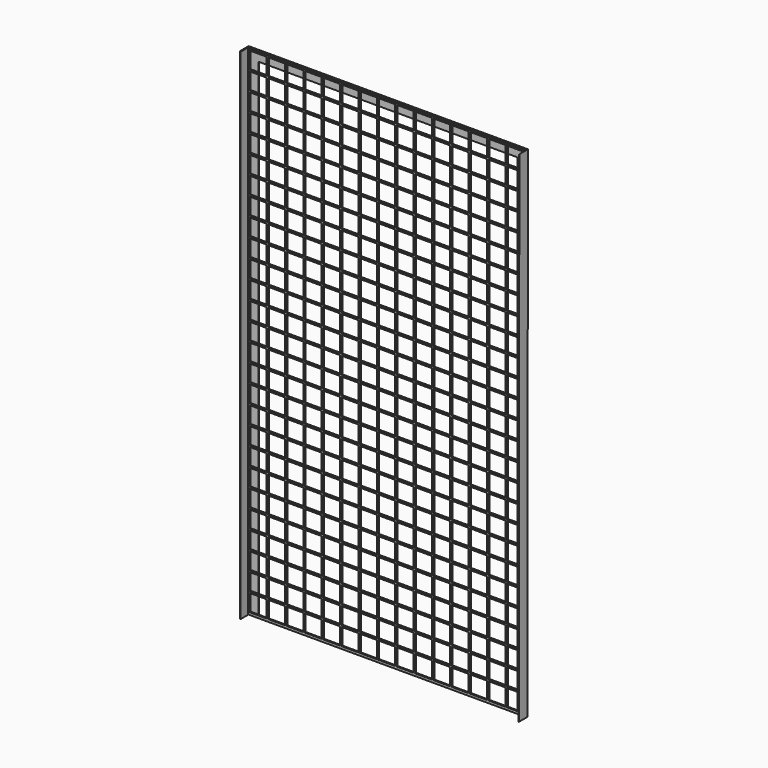
from build123d import *

# Parameters (mm, degrees)
F0_W     = 815
F0_H     = 1465
F0_W_2   = 50
F0_H_2   = 50
F1_DEPTH = 4
F3_DEPTH = 1.5
F4_DEPTH = 30


with BuildPart() as f1:
    # F0 (on Front) → F1 (new body)
    with BuildSketch(Plane.XZ):
        with Locations((407.5, -732.5)):
            Rectangle(F0_W, F0_H)
        with Locations((29, -1433)):
            Rectangle(F0_W_2, F0_H_2, mode=Mode.SUBTRACT)
        with Locations((29, -1379)):
            Rectangle(F0_W_2, F0_H_2, mode=Mode.SUBTRACT)
        with Locations((83, -1433)):
            Rectangle(F0_W_2, F0_H_2, mode=Mode.SUBTRACT)
        with Locations((83, -1379)):
            Rectangle(F0_W_2, F0_H_2, mode=Mode.SUBTRACT)
        with Locations((29, -1325)):
            Rectangle(F0_W_2, F0_H_2, mode=Mode.SUBTRACT)
        with Locations((83, -1325)):
            Rectangle(F0_W_2, F0_H_2, mode=Mode.SUBTRACT)
        with Locations((137, -1433)):
            Rectangle(F0_W_2, F0_H_2, mode=Mode.SUBTRACT)
        with Locations((137, -1379)):
            Rectangle(F0_W_2, F0_H_2, mode=Mode.SUBTRACT)
        with Locations((191, -1433)):
            Rectangle(F0_W_2, F0_H_2, mode=Mode.SUBTRACT)
        with Locations((191, -1379)):
            Rectangle(F0_W_2, F0_H_2, mode=Mode.SUBTRACT)
        with Locations((137, -1325)):
            Rectangle(F0_W_2, F0_H_2, mode=Mode.SUBTRACT)
        with Locations((191, -1325)):
            Rectangle(F0_W_2, F0_H_2, mode=Mode.SUBTRACT)
        with Locations((29, -1271)):
            Rectangle(F0_W_2, F0_H_2, mode=Mode.SUBTRACT)
        with Locations((29, -1217)):
            Rectangle(F0_W_2, F0_H_2, mode=Mode.SUBTRACT)
        with Locations((83, -1271)):
            Rectangle(F0_W_2, F0_H_2, mode=Mode.SUBTRACT)
        with Locations((83, -1217)):
            Rectangle(F0_W_2, F0_H_2, mode=Mode.SUBTRACT)
        with Locations((29, -1163)):
            Rectangle(F0_W_2, F0_H_2, mode=Mode.SUBTRACT)
        with Locations((29, -1109)):
            Rectangle(F0_W_2, F0_H_2, mode=Mode.SUBTRACT)
        with Locations((83, -1163)):
            Rectangle(F0_W_2, F0_H_2, mode=Mode.SUBTRACT)
        with Locations((83, -1109)):
            Rectangle(F0_W_2, F0_H_2, mode=Mode.SUBTRACT)
        with Locations((137, -1271)):
            Rectangle(F0_W_2, F0_H_2, mode=Mode.SUBTRACT)
        with Locations((137, -1217)):
            Rectangle(F0_W_2, F0_H_2, mode=Mode.SUBTRACT)
        with Locations((191, -1271)):
            Rectangle(F0_W_2, F0_H_2, mode=Mode.SUBTRACT)
        with Locations((191, -1217)):
            Rectangle(F0_W_2, F0_H_2, mode=Mode.SUBTRACT)
        with Locations((137, -1163)):
            Rectangle(F0_W_2, F0_H_2, mode=Mode.SUBTRACT)
        with Locations((137, -1109)):
            Rectangle(F0_W_2, F0_H_2, mode=Mode.SUBTRACT)
        with Locations((191, -1163)):
            Rectangle(F0_W_2, F0_H_2, mode=Mode.SUBTRACT)
        with Locations((191, -1109)):
            Rectangle(F0_W_2, F0_H_2, mode=Mode.SUBTRACT)
        with Locations((245, -1433)):
            Rectangle(F0_W_2, F0_H_2, mode=Mode.SUBTRACT)
        with Locations((245, -1379)):
            Rectangle(F0_W_2, F0_H_2, mode=Mode.SUBTRACT)
        with Locations((299, -1433)):
            Rectangle(F0_W_2, F0_H_2, mode=Mode.SUBTRACT)
        with Locations((299, -1379)):
            Rectangle(F0_W_2, F0_H_2, mode=Mode.SUBTRACT)
        with Locations((245, -1325)):
            Rectangle(F0_W_2, F0_H_2, mode=Mode.SUBTRACT)
        with Locations((299, -1325)):
            Rectangle(F0_W_2, F0_H_2, mode=Mode.SUBTRACT)
        with Locations((353, -1433)):
            Rectangle(F0_W_2, F0_H_2, mode=Mode.SUBTRACT)
        with Locations((353, -1379)):
            Rectangle(F0_W_2, F0_H_2, mode=Mode.SUBTRACT)
        with Locations((407, -1433)):
            Rectangle(F0_W_2, F0_H_2, mode=Mode.SUBTRACT)
        with Locations((407, -1379)):
            Rectangle(F0_W_2, F0_H_2, mode=Mode.SUBTRACT)
        with Locations((353, -1325)):
            Rectangle(F0_W_2, F0_H_2, mode=Mode.SUBTRACT)
        with Locations((407, -1325)):
            Rectangle(F0_W_2, F0_H_2, mode=Mode.SUBTRACT)
        with Locations((245, -1271)):
            Rectangle(F0_W_2, F0_H_2, mode=Mode.SUBTRACT)
        with Locations((245, -1217)):
            Rectangle(F0_W_2, F0_H_2, mode=Mode.SUBTRACT)
        with Locations((299, -1271)):
            Rectangle(F0_W_2, F0_H_2, mode=Mode.SUBTRACT)
        with Locations((299, -1217)):
            Rectangle(F0_W_2, F0_H_2, mode=Mode.SUBTRACT)
        with Locations((245, -1163)):
            Rectangle(F0_W_2, F0_H_2, mode=Mode.SUBTRACT)
        with Locations((245, -1109)):
            Rectangle(F0_W_2, F0_H_2, mode=Mode.SUBTRACT)
        with Locations((299, -1163)):
            Rectangle(F0_W_2, F0_H_2, mode=Mode.SUBTRACT)
        with Locations((299, -1109)):
            Rectangle(F0_W_2, F0_H_2, mode=Mode.SUBTRACT)
        with Locations((353, -1271)):
            Rectangle(F0_W_2, F0_H_2, mode=Mode.SUBTRACT)
        with Locations((353, -1217)):
            Rectangle(F0_W_2, F0_H_2, mode=Mode.SUBTRACT)
        with Locations((407, -1271)):
            Rectangle(F0_W_2, F0_H_2, mode=Mode.SUBTRACT)
        with Locations((407, -1217)):
            Rectangle(F0_W_2, F0_H_2, mode=Mode.SUBTRACT)
        with Locations((353, -1163)):
            Rectangle(F0_W_2, F0_H_2, mode=Mode.SUBTRACT)
        with Locations((353, -1109)):
            Rectangle(F0_W_2, F0_H_2, mode=Mode.SUBTRACT)
        with Locations((407, -1163)):
            Rectangle(F0_W_2, F0_H_2, mode=Mode.SUBTRACT)
        with Locations((407, -1109)):
            Rectangle(F0_W_2, F0_H_2, mode=Mode.SUBTRACT)
        with Locations((29, -1055)):
            Rectangle(F0_W_2, F0_H_2, mode=Mode.SUBTRACT)
        with Locations((83, -1055)):
            Rectangle(F0_W_2, F0_H_2, mode=Mode.SUBTRACT)
        with Locations((29, -1001)):
            Rectangle(F0_W_2, F0_H_2, mode=Mode.SUBTRACT)
        with Locations((29, -947)):
            Rectangle(F0_W_2, F0_H_2, mode=Mode.SUBTRACT)
        with Locations((83, -1001)):
            Rectangle(F0_W_2, F0_H_2, mode=Mode.SUBTRACT)
        with Locations((83, -947)):
            Rectangle(F0_W_2, F0_H_2, mode=Mode.SUBTRACT)
        with Locations((137, -1055)):
            Rectangle(F0_W_2, F0_H_2, mode=Mode.SUBTRACT)
        with Locations((191, -1055)):
            Rectangle(F0_W_2, F0_H_2, mode=Mode.SUBTRACT)
        with Locations((137, -1001)):
            Rectangle(F0_W_2, F0_H_2, mode=Mode.SUBTRACT)
        with Locations((137, -947)):
            Rectangle(F0_W_2, F0_H_2, mode=Mode.SUBTRACT)
        with Locations((191, -1001)):
            Rectangle(F0_W_2, F0_H_2, mode=Mode.SUBTRACT)
        with Locations((191, -947)):
            Rectangle(F0_W_2, F0_H_2, mode=Mode.SUBTRACT)
        with Locations((29, -893)):
            Rectangle(F0_W_2, F0_H_2, mode=Mode.SUBTRACT)
        with Locations((29, -839)):
            Rectangle(F0_W_2, F0_H_2, mode=Mode.SUBTRACT)
        with Locations((83, -893)):
            Rectangle(F0_W_2, F0_H_2, mode=Mode.SUBTRACT)
        with Locations((83, -839)):
            Rectangle(F0_W_2, F0_H_2, mode=Mode.SUBTRACT)
        with Locations((29, -785)):
            Rectangle(F0_W_2, F0_H_2, mode=Mode.SUBTRACT)
        with Locations((83, -785)):
            Rectangle(F0_W_2, F0_H_2, mode=Mode.SUBTRACT)
        with Locations((137, -893)):
            Rectangle(F0_W_2, F0_H_2, mode=Mode.SUBTRACT)
        with Locations((137, -839)):
            Rectangle(F0_W_2, F0_H_2, mode=Mode.SUBTRACT)
        with Locations((191, -893)):
            Rectangle(F0_W_2, F0_H_2, mode=Mode.SUBTRACT)
        with Locations((191, -839)):
            Rectangle(F0_W_2, F0_H_2, mode=Mode.SUBTRACT)
        with Locations((137, -785)):
            Rectangle(F0_W_2, F0_H_2, mode=Mode.SUBTRACT)
        with Locations((191, -785)):
            Rectangle(F0_W_2, F0_H_2, mode=Mode.SUBTRACT)
        with Locations((245, -1055)):
            Rectangle(F0_W_2, F0_H_2, mode=Mode.SUBTRACT)
        with Locations((299, -1055)):
            Rectangle(F0_W_2, F0_H_2, mode=Mode.SUBTRACT)
        with Locations((245, -1001)):
            Rectangle(F0_W_2, F0_H_2, mode=Mode.SUBTRACT)
        with Locations((245, -947)):
            Rectangle(F0_W_2, F0_H_2, mode=Mode.SUBTRACT)
        with Locations((299, -1001)):
            Rectangle(F0_W_2, F0_H_2, mode=Mode.SUBTRACT)
        with Locations((299, -947)):
            Rectangle(F0_W_2, F0_H_2, mode=Mode.SUBTRACT)
        with Locations((353, -1055)):
            Rectangle(F0_W_2, F0_H_2, mode=Mode.SUBTRACT)
        with Locations((407, -1055)):
            Rectangle(F0_W_2, F0_H_2, mode=Mode.SUBTRACT)
        with Locations((353, -1001)):
            Rectangle(F0_W_2, F0_H_2, mode=Mode.SUBTRACT)
        with Locations((353, -947)):
            Rectangle(F0_W_2, F0_H_2, mode=Mode.SUBTRACT)
        with Locations((407, -1001)):
            Rectangle(F0_W_2, F0_H_2, mode=Mode.SUBTRACT)
        with Locations((407, -947)):
            Rectangle(F0_W_2, F0_H_2, mode=Mode.SUBTRACT)
        with Locations((245, -893)):
            Rectangle(F0_W_2, F0_H_2, mode=Mode.SUBTRACT)
        with Locations((245, -839)):
            Rectangle(F0_W_2, F0_H_2, mode=Mode.SUBTRACT)
        with Locations((299, -893)):
            Rectangle(F0_W_2, F0_H_2, mode=Mode.SUBTRACT)
        with Locations((299, -839)):
            Rectangle(F0_W_2, F0_H_2, mode=Mode.SUBTRACT)
        with Locations((245, -785)):
            Rectangle(F0_W_2, F0_H_2, mode=Mode.SUBTRACT)
        with Locations((299, -785)):
            Rectangle(F0_W_2, F0_H_2, mode=Mode.SUBTRACT)
        with Locations((353, -893)):
            Rectangle(F0_W_2, F0_H_2, mode=Mode.SUBTRACT)
        with Locations((353, -839)):
            Rectangle(F0_W_2, F0_H_2, mode=Mode.SUBTRACT)
        with Locations((407, -893)):
            Rectangle(F0_W_2, F0_H_2, mode=Mode.SUBTRACT)
        with Locations((407, -839)):
            Rectangle(F0_W_2, F0_H_2, mode=Mode.SUBTRACT)
        with Locations((353, -785)):
            Rectangle(F0_W_2, F0_H_2, mode=Mode.SUBTRACT)
        with Locations((407, -785)):
            Rectangle(F0_W_2, F0_H_2, mode=Mode.SUBTRACT)
        with Locations((461, -1433)):
            Rectangle(F0_W_2, F0_H_2, mode=Mode.SUBTRACT)
        with Locations((461, -1379)):
            Rectangle(F0_W_2, F0_H_2, mode=Mode.SUBTRACT)
        with Locations((461, -1325)):
            Rectangle(F0_W_2, F0_H_2, mode=Mode.SUBTRACT)
        with Locations((515, -1433)):
            Rectangle(F0_W_2, F0_H_2, mode=Mode.SUBTRACT)
        with Locations((515, -1379)):
            Rectangle(F0_W_2, F0_H_2, mode=Mode.SUBTRACT)
        with Locations((569, -1433)):
            Rectangle(F0_W_2, F0_H_2, mode=Mode.SUBTRACT)
        with Locations((569, -1379)):
            Rectangle(F0_W_2, F0_H_2, mode=Mode.SUBTRACT)
        with Locations((515, -1325)):
            Rectangle(F0_W_2, F0_H_2, mode=Mode.SUBTRACT)
        with Locations((569, -1325)):
            Rectangle(F0_W_2, F0_H_2, mode=Mode.SUBTRACT)
        with Locations((461, -1271)):
            Rectangle(F0_W_2, F0_H_2, mode=Mode.SUBTRACT)
        with Locations((461, -1217)):
            Rectangle(F0_W_2, F0_H_2, mode=Mode.SUBTRACT)
        with Locations((461, -1163)):
            Rectangle(F0_W_2, F0_H_2, mode=Mode.SUBTRACT)
        with Locations((461, -1109)):
            Rectangle(F0_W_2, F0_H_2, mode=Mode.SUBTRACT)
        with Locations((515, -1271)):
            Rectangle(F0_W_2, F0_H_2, mode=Mode.SUBTRACT)
        with Locations((515, -1217)):
            Rectangle(F0_W_2, F0_H_2, mode=Mode.SUBTRACT)
        with Locations((569, -1271)):
            Rectangle(F0_W_2, F0_H_2, mode=Mode.SUBTRACT)
        with Locations((569, -1217)):
            Rectangle(F0_W_2, F0_H_2, mode=Mode.SUBTRACT)
        with Locations((515, -1163)):
            Rectangle(F0_W_2, F0_H_2, mode=Mode.SUBTRACT)
        with Locations((515, -1109)):
            Rectangle(F0_W_2, F0_H_2, mode=Mode.SUBTRACT)
        with Locations((569, -1163)):
            Rectangle(F0_W_2, F0_H_2, mode=Mode.SUBTRACT)
        with Locations((569, -1109)):
            Rectangle(F0_W_2, F0_H_2, mode=Mode.SUBTRACT)
        with Locations((623, -1433)):
            Rectangle(F0_W_2, F0_H_2, mode=Mode.SUBTRACT)
        with Locations((623, -1379)):
            Rectangle(F0_W_2, F0_H_2, mode=Mode.SUBTRACT)
        with Locations((677, -1433)):
            Rectangle(F0_W_2, F0_H_2, mode=Mode.SUBTRACT)
        with Locations((677, -1379)):
            Rectangle(F0_W_2, F0_H_2, mode=Mode.SUBTRACT)
        with Locations((623, -1325)):
            Rectangle(F0_W_2, F0_H_2, mode=Mode.SUBTRACT)
        with Locations((677, -1325)):
            Rectangle(F0_W_2, F0_H_2, mode=Mode.SUBTRACT)
        with Locations((731, -1433)):
            Rectangle(F0_W_2, F0_H_2, mode=Mode.SUBTRACT)
        with Locations((731, -1379)):
            Rectangle(F0_W_2, F0_H_2, mode=Mode.SUBTRACT)
        with Locations((785, -1433)):
            Rectangle(F0_W_2, F0_H_2, mode=Mode.SUBTRACT)
        with Locations((785, -1379)):
            Rectangle(F0_W_2, F0_H_2, mode=Mode.SUBTRACT)
        with Locations((731, -1325)):
            Rectangle(F0_W_2, F0_H_2, mode=Mode.SUBTRACT)
        with Locations((785, -1325)):
            Rectangle(F0_W_2, F0_H_2, mode=Mode.SUBTRACT)
        with Locations((623, -1271)):
            Rectangle(F0_W_2, F0_H_2, mode=Mode.SUBTRACT)
        with Locations((623, -1217)):
            Rectangle(F0_W_2, F0_H_2, mode=Mode.SUBTRACT)
        with Locations((677, -1271)):
            Rectangle(F0_W_2, F0_H_2, mode=Mode.SUBTRACT)
        with Locations((677, -1217)):
            Rectangle(F0_W_2, F0_H_2, mode=Mode.SUBTRACT)
        with Locations((623, -1163)):
            Rectangle(F0_W_2, F0_H_2, mode=Mode.SUBTRACT)
        with Locations((623, -1109)):
            Rectangle(F0_W_2, F0_H_2, mode=Mode.SUBTRACT)
        with Locations((677, -1163)):
            Rectangle(F0_W_2, F0_H_2, mode=Mode.SUBTRACT)
        with Locations((677, -1109)):
            Rectangle(F0_W_2, F0_H_2, mode=Mode.SUBTRACT)
        with Locations((731, -1271)):
            Rectangle(F0_W_2, F0_H_2, mode=Mode.SUBTRACT)
        with Locations((731, -1217)):
            Rectangle(F0_W_2, F0_H_2, mode=Mode.SUBTRACT)
        with Locations((785, -1271)):
            Rectangle(F0_W_2, F0_H_2, mode=Mode.SUBTRACT)
        with Locations((785, -1217)):
            Rectangle(F0_W_2, F0_H_2, mode=Mode.SUBTRACT)
        with Locations((731, -1163)):
            Rectangle(F0_W_2, F0_H_2, mode=Mode.SUBTRACT)
        with Locations((731, -1109)):
            Rectangle(F0_W_2, F0_H_2, mode=Mode.SUBTRACT)
        with Locations((785, -1163)):
            Rectangle(F0_W_2, F0_H_2, mode=Mode.SUBTRACT)
        with Locations((785, -1109)):
            Rectangle(F0_W_2, F0_H_2, mode=Mode.SUBTRACT)
        with Locations((461, -1055)):
            Rectangle(F0_W_2, F0_H_2, mode=Mode.SUBTRACT)
        with Locations((461, -1001)):
            Rectangle(F0_W_2, F0_H_2, mode=Mode.SUBTRACT)
        with Locations((461, -947)):
            Rectangle(F0_W_2, F0_H_2, mode=Mode.SUBTRACT)
        with Locations((515, -1055)):
            Rectangle(F0_W_2, F0_H_2, mode=Mode.SUBTRACT)
        with Locations((569, -1055)):
            Rectangle(F0_W_2, F0_H_2, mode=Mode.SUBTRACT)
        with Locations((515, -1001)):
            Rectangle(F0_W_2, F0_H_2, mode=Mode.SUBTRACT)
        with Locations((515, -947)):
            Rectangle(F0_W_2, F0_H_2, mode=Mode.SUBTRACT)
        with Locations((569, -1001)):
            Rectangle(F0_W_2, F0_H_2, mode=Mode.SUBTRACT)
        with Locations((569, -947)):
            Rectangle(F0_W_2, F0_H_2, mode=Mode.SUBTRACT)
        with Locations((461, -893)):
            Rectangle(F0_W_2, F0_H_2, mode=Mode.SUBTRACT)
        with Locations((461, -839)):
            Rectangle(F0_W_2, F0_H_2, mode=Mode.SUBTRACT)
        with Locations((461, -785)):
            Rectangle(F0_W_2, F0_H_2, mode=Mode.SUBTRACT)
        with Locations((515, -893)):
            Rectangle(F0_W_2, F0_H_2, mode=Mode.SUBTRACT)
        with Locations((515, -839)):
            Rectangle(F0_W_2, F0_H_2, mode=Mode.SUBTRACT)
        with Locations((569, -893)):
            Rectangle(F0_W_2, F0_H_2, mode=Mode.SUBTRACT)
        with Locations((569, -839)):
            Rectangle(F0_W_2, F0_H_2, mode=Mode.SUBTRACT)
        with Locations((515, -785)):
            Rectangle(F0_W_2, F0_H_2, mode=Mode.SUBTRACT)
        with Locations((569, -785)):
            Rectangle(F0_W_2, F0_H_2, mode=Mode.SUBTRACT)
        with Locations((623, -1055)):
            Rectangle(F0_W_2, F0_H_2, mode=Mode.SUBTRACT)
        with Locations((677, -1055)):
            Rectangle(F0_W_2, F0_H_2, mode=Mode.SUBTRACT)
        with Locations((623, -1001)):
            Rectangle(F0_W_2, F0_H_2, mode=Mode.SUBTRACT)
        with Locations((623, -947)):
            Rectangle(F0_W_2, F0_H_2, mode=Mode.SUBTRACT)
        with Locations((677, -1001)):
            Rectangle(F0_W_2, F0_H_2, mode=Mode.SUBTRACT)
        with Locations((677, -947)):
            Rectangle(F0_W_2, F0_H_2, mode=Mode.SUBTRACT)
        with Locations((731, -1055)):
            Rectangle(F0_W_2, F0_H_2, mode=Mode.SUBTRACT)
        with Locations((785, -1055)):
            Rectangle(F0_W_2, F0_H_2, mode=Mode.SUBTRACT)
        with Locations((731, -1001)):
            Rectangle(F0_W_2, F0_H_2, mode=Mode.SUBTRACT)
        with Locations((731, -947)):
            Rectangle(F0_W_2, F0_H_2, mode=Mode.SUBTRACT)
        with Locations((785, -1001)):
            Rectangle(F0_W_2, F0_H_2, mode=Mode.SUBTRACT)
        with Locations((785, -947)):
            Rectangle(F0_W_2, F0_H_2, mode=Mode.SUBTRACT)
        with Locations((623, -893)):
            Rectangle(F0_W_2, F0_H_2, mode=Mode.SUBTRACT)
        with Locations((623, -839)):
            Rectangle(F0_W_2, F0_H_2, mode=Mode.SUBTRACT)
        with Locations((677, -893)):
            Rectangle(F0_W_2, F0_H_2, mode=Mode.SUBTRACT)
        with Locations((677, -839)):
            Rectangle(F0_W_2, F0_H_2, mode=Mode.SUBTRACT)
        with Locations((623, -785)):
            Rectangle(F0_W_2, F0_H_2, mode=Mode.SUBTRACT)
        with Locations((677, -785)):
            Rectangle(F0_W_2, F0_H_2, mode=Mode.SUBTRACT)
        with Locations((731, -893)):
            Rectangle(F0_W_2, F0_H_2, mode=Mode.SUBTRACT)
        with Locations((731, -839)):
            Rectangle(F0_W_2, F0_H_2, mode=Mode.SUBTRACT)
        with Locations((785, -893)):
            Rectangle(F0_W_2, F0_H_2, mode=Mode.SUBTRACT)
        with Locations((785, -839)):
            Rectangle(F0_W_2, F0_H_2, mode=Mode.SUBTRACT)
        with Locations((731, -785)):
            Rectangle(F0_W_2, F0_H_2, mode=Mode.SUBTRACT)
        with Locations((785, -785)):
            Rectangle(F0_W_2, F0_H_2, mode=Mode.SUBTRACT)
        with Locations((29, -731)):
            Rectangle(F0_W_2, F0_H_2, mode=Mode.SUBTRACT)
        with Locations((29, -677)):
            Rectangle(F0_W_2, F0_H_2, mode=Mode.SUBTRACT)
        with Locations((83, -731)):
            Rectangle(F0_W_2, F0_H_2, mode=Mode.SUBTRACT)
        with Locations((83, -677)):
            Rectangle(F0_W_2, F0_H_2, mode=Mode.SUBTRACT)
        with Locations((29, -623)):
            Rectangle(F0_W_2, F0_H_2, mode=Mode.SUBTRACT)
        with Locations((29, -569)):
            Rectangle(F0_W_2, F0_H_2, mode=Mode.SUBTRACT)
        with Locations((83, -623)):
            Rectangle(F0_W_2, F0_H_2, mode=Mode.SUBTRACT)
        with Locations((83, -569)):
            Rectangle(F0_W_2, F0_H_2, mode=Mode.SUBTRACT)
        with Locations((137, -731)):
            Rectangle(F0_W_2, F0_H_2, mode=Mode.SUBTRACT)
        with Locations((137, -677)):
            Rectangle(F0_W_2, F0_H_2, mode=Mode.SUBTRACT)
        with Locations((191, -731)):
            Rectangle(F0_W_2, F0_H_2, mode=Mode.SUBTRACT)
        with Locations((191, -677)):
            Rectangle(F0_W_2, F0_H_2, mode=Mode.SUBTRACT)
        with Locations((137, -623)):
            Rectangle(F0_W_2, F0_H_2, mode=Mode.SUBTRACT)
        with Locations((137, -569)):
            Rectangle(F0_W_2, F0_H_2, mode=Mode.SUBTRACT)
        with Locations((191, -623)):
            Rectangle(F0_W_2, F0_H_2, mode=Mode.SUBTRACT)
        with Locations((191, -569)):
            Rectangle(F0_W_2, F0_H_2, mode=Mode.SUBTRACT)
        with Locations((29, -515)):
            Rectangle(F0_W_2, F0_H_2, mode=Mode.SUBTRACT)
        with Locations((29, -461)):
            Rectangle(F0_W_2, F0_H_2, mode=Mode.SUBTRACT)
        with Locations((83, -515)):
            Rectangle(F0_W_2, F0_H_2, mode=Mode.SUBTRACT)
        with Locations((83, -461)):
            Rectangle(F0_W_2, F0_H_2, mode=Mode.SUBTRACT)
        with Locations((29, -407)):
            Rectangle(F0_W_2, F0_H_2, mode=Mode.SUBTRACT)
        with Locations((83, -407)):
            Rectangle(F0_W_2, F0_H_2, mode=Mode.SUBTRACT)
        with Locations((137, -515)):
            Rectangle(F0_W_2, F0_H_2, mode=Mode.SUBTRACT)
        with Locations((137, -461)):
            Rectangle(F0_W_2, F0_H_2, mode=Mode.SUBTRACT)
        with Locations((191, -515)):
            Rectangle(F0_W_2, F0_H_2, mode=Mode.SUBTRACT)
        with Locations((191, -461)):
            Rectangle(F0_W_2, F0_H_2, mode=Mode.SUBTRACT)
        with Locations((137, -407)):
            Rectangle(F0_W_2, F0_H_2, mode=Mode.SUBTRACT)
        with Locations((191, -407)):
            Rectangle(F0_W_2, F0_H_2, mode=Mode.SUBTRACT)
        with Locations((245, -731)):
            Rectangle(F0_W_2, F0_H_2, mode=Mode.SUBTRACT)
        with Locations((245, -677)):
            Rectangle(F0_W_2, F0_H_2, mode=Mode.SUBTRACT)
        with Locations((299, -731)):
            Rectangle(F0_W_2, F0_H_2, mode=Mode.SUBTRACT)
        with Locations((299, -677)):
            Rectangle(F0_W_2, F0_H_2, mode=Mode.SUBTRACT)
        with Locations((245, -623)):
            Rectangle(F0_W_2, F0_H_2, mode=Mode.SUBTRACT)
        with Locations((245, -569)):
            Rectangle(F0_W_2, F0_H_2, mode=Mode.SUBTRACT)
        with Locations((299, -623)):
            Rectangle(F0_W_2, F0_H_2, mode=Mode.SUBTRACT)
        with Locations((299, -569)):
            Rectangle(F0_W_2, F0_H_2, mode=Mode.SUBTRACT)
        with Locations((353, -731)):
            Rectangle(F0_W_2, F0_H_2, mode=Mode.SUBTRACT)
        with Locations((353, -677)):
            Rectangle(F0_W_2, F0_H_2, mode=Mode.SUBTRACT)
        with Locations((407, -731)):
            Rectangle(F0_W_2, F0_H_2, mode=Mode.SUBTRACT)
        with Locations((407, -677)):
            Rectangle(F0_W_2, F0_H_2, mode=Mode.SUBTRACT)
        with Locations((353, -623)):
            Rectangle(F0_W_2, F0_H_2, mode=Mode.SUBTRACT)
        with Locations((353, -569)):
            Rectangle(F0_W_2, F0_H_2, mode=Mode.SUBTRACT)
        with Locations((407, -623)):
            Rectangle(F0_W_2, F0_H_2, mode=Mode.SUBTRACT)
        with Locations((407, -569)):
            Rectangle(F0_W_2, F0_H_2, mode=Mode.SUBTRACT)
        with Locations((245, -515)):
            Rectangle(F0_W_2, F0_H_2, mode=Mode.SUBTRACT)
        with Locations((245, -461)):
            Rectangle(F0_W_2, F0_H_2, mode=Mode.SUBTRACT)
        with Locations((299, -515)):
            Rectangle(F0_W_2, F0_H_2, mode=Mode.SUBTRACT)
        with Locations((299, -461)):
            Rectangle(F0_W_2, F0_H_2, mode=Mode.SUBTRACT)
        with Locations((245, -407)):
            Rectangle(F0_W_2, F0_H_2, mode=Mode.SUBTRACT)
        with Locations((299, -407)):
            Rectangle(F0_W_2, F0_H_2, mode=Mode.SUBTRACT)
        with Locations((353, -515)):
            Rectangle(F0_W_2, F0_H_2, mode=Mode.SUBTRACT)
        with Locations((353, -461)):
            Rectangle(F0_W_2, F0_H_2, mode=Mode.SUBTRACT)
        with Locations((407, -515)):
            Rectangle(F0_W_2, F0_H_2, mode=Mode.SUBTRACT)
        with Locations((407, -461)):
            Rectangle(F0_W_2, F0_H_2, mode=Mode.SUBTRACT)
        with Locations((353, -407)):
            Rectangle(F0_W_2, F0_H_2, mode=Mode.SUBTRACT)
        with Locations((407, -407)):
            Rectangle(F0_W_2, F0_H_2, mode=Mode.SUBTRACT)
        with Locations((29, -353)):
            Rectangle(F0_W_2, F0_H_2, mode=Mode.SUBTRACT)
        with Locations((29, -299)):
            Rectangle(F0_W_2, F0_H_2, mode=Mode.SUBTRACT)
        with Locations((83, -353)):
            Rectangle(F0_W_2, F0_H_2, mode=Mode.SUBTRACT)
        with Locations((83, -299)):
            Rectangle(F0_W_2, F0_H_2, mode=Mode.SUBTRACT)
        with Locations((29, -245)):
            Rectangle(F0_W_2, F0_H_2, mode=Mode.SUBTRACT)
        with Locations((29, -191)):
            Rectangle(F0_W_2, F0_H_2, mode=Mode.SUBTRACT)
        with Locations((83, -245)):
            Rectangle(F0_W_2, F0_H_2, mode=Mode.SUBTRACT)
        with Locations((83, -191)):
            Rectangle(F0_W_2, F0_H_2, mode=Mode.SUBTRACT)
        with Locations((137, -353)):
            Rectangle(F0_W_2, F0_H_2, mode=Mode.SUBTRACT)
        with Locations((137, -299)):
            Rectangle(F0_W_2, F0_H_2, mode=Mode.SUBTRACT)
        with Locations((191, -353)):
            Rectangle(F0_W_2, F0_H_2, mode=Mode.SUBTRACT)
        with Locations((191, -299)):
            Rectangle(F0_W_2, F0_H_2, mode=Mode.SUBTRACT)
        with Locations((137, -245)):
            Rectangle(F0_W_2, F0_H_2, mode=Mode.SUBTRACT)
        with Locations((137, -191)):
            Rectangle(F0_W_2, F0_H_2, mode=Mode.SUBTRACT)
        with Locations((191, -245)):
            Rectangle(F0_W_2, F0_H_2, mode=Mode.SUBTRACT)
        with Locations((191, -191)):
            Rectangle(F0_W_2, F0_H_2, mode=Mode.SUBTRACT)
        with Locations((29, -137)):
            Rectangle(F0_W_2, F0_H_2, mode=Mode.SUBTRACT)
        with Locations((83, -137)):
            Rectangle(F0_W_2, F0_H_2, mode=Mode.SUBTRACT)
        with Locations((29, -83)):
            Rectangle(F0_W_2, F0_H_2, mode=Mode.SUBTRACT)
        with Locations((29, -29)):
            Rectangle(F0_W_2, F0_H_2, mode=Mode.SUBTRACT)
        with Locations((83, -83)):
            Rectangle(F0_W_2, F0_H_2, mode=Mode.SUBTRACT)
        with Locations((83, -29)):
            Rectangle(F0_W_2, F0_H_2, mode=Mode.SUBTRACT)
        with Locations((137, -137)):
            Rectangle(F0_W_2, F0_H_2, mode=Mode.SUBTRACT)
        with Locations((191, -137)):
            Rectangle(F0_W_2, F0_H_2, mode=Mode.SUBTRACT)
        with Locations((137, -83)):
            Rectangle(F0_W_2, F0_H_2, mode=Mode.SUBTRACT)
        with Locations((137, -29)):
            Rectangle(F0_W_2, F0_H_2, mode=Mode.SUBTRACT)
        with Locations((191, -83)):
            Rectangle(F0_W_2, F0_H_2, mode=Mode.SUBTRACT)
        with Locations((191, -29)):
            Rectangle(F0_W_2, F0_H_2, mode=Mode.SUBTRACT)
        with Locations((245, -353)):
            Rectangle(F0_W_2, F0_H_2, mode=Mode.SUBTRACT)
        with Locations((245, -299)):
            Rectangle(F0_W_2, F0_H_2, mode=Mode.SUBTRACT)
        with Locations((299, -353)):
            Rectangle(F0_W_2, F0_H_2, mode=Mode.SUBTRACT)
        with Locations((299, -299)):
            Rectangle(F0_W_2, F0_H_2, mode=Mode.SUBTRACT)
        with Locations((245, -245)):
            Rectangle(F0_W_2, F0_H_2, mode=Mode.SUBTRACT)
        with Locations((245, -191)):
            Rectangle(F0_W_2, F0_H_2, mode=Mode.SUBTRACT)
        with Locations((299, -245)):
            Rectangle(F0_W_2, F0_H_2, mode=Mode.SUBTRACT)
        with Locations((299, -191)):
            Rectangle(F0_W_2, F0_H_2, mode=Mode.SUBTRACT)
        with Locations((353, -353)):
            Rectangle(F0_W_2, F0_H_2, mode=Mode.SUBTRACT)
        with Locations((353, -299)):
            Rectangle(F0_W_2, F0_H_2, mode=Mode.SUBTRACT)
        with Locations((407, -353)):
            Rectangle(F0_W_2, F0_H_2, mode=Mode.SUBTRACT)
        with Locations((407, -299)):
            Rectangle(F0_W_2, F0_H_2, mode=Mode.SUBTRACT)
        with Locations((353, -245)):
            Rectangle(F0_W_2, F0_H_2, mode=Mode.SUBTRACT)
        with Locations((353, -191)):
            Rectangle(F0_W_2, F0_H_2, mode=Mode.SUBTRACT)
        with Locations((407, -245)):
            Rectangle(F0_W_2, F0_H_2, mode=Mode.SUBTRACT)
        with Locations((407, -191)):
            Rectangle(F0_W_2, F0_H_2, mode=Mode.SUBTRACT)
        with Locations((245, -137)):
            Rectangle(F0_W_2, F0_H_2, mode=Mode.SUBTRACT)
        with Locations((299, -137)):
            Rectangle(F0_W_2, F0_H_2, mode=Mode.SUBTRACT)
        with Locations((245, -83)):
            Rectangle(F0_W_2, F0_H_2, mode=Mode.SUBTRACT)
        with Locations((245, -29)):
            Rectangle(F0_W_2, F0_H_2, mode=Mode.SUBTRACT)
        with Locations((299, -83)):
            Rectangle(F0_W_2, F0_H_2, mode=Mode.SUBTRACT)
        with Locations((299, -29)):
            Rectangle(F0_W_2, F0_H_2, mode=Mode.SUBTRACT)
        with Locations((353, -137)):
            Rectangle(F0_W_2, F0_H_2, mode=Mode.SUBTRACT)
        with Locations((407, -137)):
            Rectangle(F0_W_2, F0_H_2, mode=Mode.SUBTRACT)
        with Locations((353, -83)):
            Rectangle(F0_W_2, F0_H_2, mode=Mode.SUBTRACT)
        with Locations((353, -29)):
            Rectangle(F0_W_2, F0_H_2, mode=Mode.SUBTRACT)
        with Locations((407, -83)):
            Rectangle(F0_W_2, F0_H_2, mode=Mode.SUBTRACT)
        with Locations((407, -29)):
            Rectangle(F0_W_2, F0_H_2, mode=Mode.SUBTRACT)
        with Locations((461, -731)):
            Rectangle(F0_W_2, F0_H_2, mode=Mode.SUBTRACT)
        with Locations((461, -677)):
            Rectangle(F0_W_2, F0_H_2, mode=Mode.SUBTRACT)
        with Locations((461, -623)):
            Rectangle(F0_W_2, F0_H_2, mode=Mode.SUBTRACT)
        with Locations((461, -569)):
            Rectangle(F0_W_2, F0_H_2, mode=Mode.SUBTRACT)
        with Locations((515, -731)):
            Rectangle(F0_W_2, F0_H_2, mode=Mode.SUBTRACT)
        with Locations((515, -677)):
            Rectangle(F0_W_2, F0_H_2, mode=Mode.SUBTRACT)
        with Locations((569, -731)):
            Rectangle(F0_W_2, F0_H_2, mode=Mode.SUBTRACT)
        with Locations((569, -677)):
            Rectangle(F0_W_2, F0_H_2, mode=Mode.SUBTRACT)
        with Locations((515, -623)):
            Rectangle(F0_W_2, F0_H_2, mode=Mode.SUBTRACT)
        with Locations((515, -569)):
            Rectangle(F0_W_2, F0_H_2, mode=Mode.SUBTRACT)
        with Locations((569, -623)):
            Rectangle(F0_W_2, F0_H_2, mode=Mode.SUBTRACT)
        with Locations((569, -569)):
            Rectangle(F0_W_2, F0_H_2, mode=Mode.SUBTRACT)
        with Locations((461, -515)):
            Rectangle(F0_W_2, F0_H_2, mode=Mode.SUBTRACT)
        with Locations((461, -461)):
            Rectangle(F0_W_2, F0_H_2, mode=Mode.SUBTRACT)
        with Locations((461, -407)):
            Rectangle(F0_W_2, F0_H_2, mode=Mode.SUBTRACT)
        with Locations((515, -515)):
            Rectangle(F0_W_2, F0_H_2, mode=Mode.SUBTRACT)
        with Locations((515, -461)):
            Rectangle(F0_W_2, F0_H_2, mode=Mode.SUBTRACT)
        with Locations((569, -515)):
            Rectangle(F0_W_2, F0_H_2, mode=Mode.SUBTRACT)
        with Locations((569, -461)):
            Rectangle(F0_W_2, F0_H_2, mode=Mode.SUBTRACT)
        with Locations((515, -407)):
            Rectangle(F0_W_2, F0_H_2, mode=Mode.SUBTRACT)
        with Locations((569, -407)):
            Rectangle(F0_W_2, F0_H_2, mode=Mode.SUBTRACT)
        with Locations((623, -731)):
            Rectangle(F0_W_2, F0_H_2, mode=Mode.SUBTRACT)
        with Locations((623, -677)):
            Rectangle(F0_W_2, F0_H_2, mode=Mode.SUBTRACT)
        with Locations((677, -731)):
            Rectangle(F0_W_2, F0_H_2, mode=Mode.SUBTRACT)
        with Locations((677, -677)):
            Rectangle(F0_W_2, F0_H_2, mode=Mode.SUBTRACT)
        with Locations((623, -623)):
            Rectangle(F0_W_2, F0_H_2, mode=Mode.SUBTRACT)
        with Locations((623, -569)):
            Rectangle(F0_W_2, F0_H_2, mode=Mode.SUBTRACT)
        with Locations((677, -623)):
            Rectangle(F0_W_2, F0_H_2, mode=Mode.SUBTRACT)
        with Locations((677, -569)):
            Rectangle(F0_W_2, F0_H_2, mode=Mode.SUBTRACT)
        with Locations((731, -731)):
            Rectangle(F0_W_2, F0_H_2, mode=Mode.SUBTRACT)
        with Locations((731, -677)):
            Rectangle(F0_W_2, F0_H_2, mode=Mode.SUBTRACT)
        with Locations((785, -731)):
            Rectangle(F0_W_2, F0_H_2, mode=Mode.SUBTRACT)
        with Locations((785, -677)):
            Rectangle(F0_W_2, F0_H_2, mode=Mode.SUBTRACT)
        with Locations((731, -623)):
            Rectangle(F0_W_2, F0_H_2, mode=Mode.SUBTRACT)
        with Locations((731, -569)):
            Rectangle(F0_W_2, F0_H_2, mode=Mode.SUBTRACT)
        with Locations((785, -623)):
            Rectangle(F0_W_2, F0_H_2, mode=Mode.SUBTRACT)
        with Locations((785, -569)):
            Rectangle(F0_W_2, F0_H_2, mode=Mode.SUBTRACT)
        with Locations((623, -515)):
            Rectangle(F0_W_2, F0_H_2, mode=Mode.SUBTRACT)
        with Locations((623, -461)):
            Rectangle(F0_W_2, F0_H_2, mode=Mode.SUBTRACT)
        with Locations((677, -515)):
            Rectangle(F0_W_2, F0_H_2, mode=Mode.SUBTRACT)
        with Locations((677, -461)):
            Rectangle(F0_W_2, F0_H_2, mode=Mode.SUBTRACT)
        with Locations((623, -407)):
            Rectangle(F0_W_2, F0_H_2, mode=Mode.SUBTRACT)
        with Locations((677, -407)):
            Rectangle(F0_W_2, F0_H_2, mode=Mode.SUBTRACT)
        with Locations((731, -515)):
            Rectangle(F0_W_2, F0_H_2, mode=Mode.SUBTRACT)
        with Locations((731, -461)):
            Rectangle(F0_W_2, F0_H_2, mode=Mode.SUBTRACT)
        with Locations((785, -515)):
            Rectangle(F0_W_2, F0_H_2, mode=Mode.SUBTRACT)
        with Locations((785, -461)):
            Rectangle(F0_W_2, F0_H_2, mode=Mode.SUBTRACT)
        with Locations((731, -407)):
            Rectangle(F0_W_2, F0_H_2, mode=Mode.SUBTRACT)
        with Locations((785, -407)):
            Rectangle(F0_W_2, F0_H_2, mode=Mode.SUBTRACT)
        with Locations((461, -353)):
            Rectangle(F0_W_2, F0_H_2, mode=Mode.SUBTRACT)
        with Locations((461, -299)):
            Rectangle(F0_W_2, F0_H_2, mode=Mode.SUBTRACT)
        with Locations((461, -245)):
            Rectangle(F0_W_2, F0_H_2, mode=Mode.SUBTRACT)
        with Locations((461, -191)):
            Rectangle(F0_W_2, F0_H_2, mode=Mode.SUBTRACT)
        with Locations((515, -353)):
            Rectangle(F0_W_2, F0_H_2, mode=Mode.SUBTRACT)
        with Locations((515, -299)):
            Rectangle(F0_W_2, F0_H_2, mode=Mode.SUBTRACT)
        with Locations((569, -353)):
            Rectangle(F0_W_2, F0_H_2, mode=Mode.SUBTRACT)
        with Locations((569, -299)):
            Rectangle(F0_W_2, F0_H_2, mode=Mode.SUBTRACT)
        with Locations((515, -245)):
            Rectangle(F0_W_2, F0_H_2, mode=Mode.SUBTRACT)
        with Locations((515, -191)):
            Rectangle(F0_W_2, F0_H_2, mode=Mode.SUBTRACT)
        with Locations((569, -245)):
            Rectangle(F0_W_2, F0_H_2, mode=Mode.SUBTRACT)
        with Locations((569, -191)):
            Rectangle(F0_W_2, F0_H_2, mode=Mode.SUBTRACT)
        with Locations((461, -137)):
            Rectangle(F0_W_2, F0_H_2, mode=Mode.SUBTRACT)
        with Locations((461, -83)):
            Rectangle(F0_W_2, F0_H_2, mode=Mode.SUBTRACT)
        with Locations((461, -29)):
            Rectangle(F0_W_2, F0_H_2, mode=Mode.SUBTRACT)
        with Locations((515, -137)):
            Rectangle(F0_W_2, F0_H_2, mode=Mode.SUBTRACT)
        with Locations((569, -137)):
            Rectangle(F0_W_2, F0_H_2, mode=Mode.SUBTRACT)
        with Locations((515, -83)):
            Rectangle(F0_W_2, F0_H_2, mode=Mode.SUBTRACT)
        with Locations((515, -29)):
            Rectangle(F0_W_2, F0_H_2, mode=Mode.SUBTRACT)
        with Locations((569, -83)):
            Rectangle(F0_W_2, F0_H_2, mode=Mode.SUBTRACT)
        with Locations((569, -29)):
            Rectangle(F0_W_2, F0_H_2, mode=Mode.SUBTRACT)
        with Locations((623, -353)):
            Rectangle(F0_W_2, F0_H_2, mode=Mode.SUBTRACT)
        with Locations((623, -299)):
            Rectangle(F0_W_2, F0_H_2, mode=Mode.SUBTRACT)
        with Locations((677, -353)):
            Rectangle(F0_W_2, F0_H_2, mode=Mode.SUBTRACT)
        with Locations((677, -299)):
            Rectangle(F0_W_2, F0_H_2, mode=Mode.SUBTRACT)
        with Locations((623, -245)):
            Rectangle(F0_W_2, F0_H_2, mode=Mode.SUBTRACT)
        with Locations((623, -191)):
            Rectangle(F0_W_2, F0_H_2, mode=Mode.SUBTRACT)
        with Locations((677, -245)):
            Rectangle(F0_W_2, F0_H_2, mode=Mode.SUBTRACT)
        with Locations((677, -191)):
            Rectangle(F0_W_2, F0_H_2, mode=Mode.SUBTRACT)
        with Locations((731, -353)):
            Rectangle(F0_W_2, F0_H_2, mode=Mode.SUBTRACT)
        with Locations((731, -299)):
            Rectangle(F0_W_2, F0_H_2, mode=Mode.SUBTRACT)
        with Locations((785, -353)):
            Rectangle(F0_W_2, F0_H_2, mode=Mode.SUBTRACT)
        with Locations((785, -299)):
            Rectangle(F0_W_2, F0_H_2, mode=Mode.SUBTRACT)
        with Locations((731, -245)):
            Rectangle(F0_W_2, F0_H_2, mode=Mode.SUBTRACT)
        with Locations((731, -191)):
            Rectangle(F0_W_2, F0_H_2, mode=Mode.SUBTRACT)
        with Locations((785, -245)):
            Rectangle(F0_W_2, F0_H_2, mode=Mode.SUBTRACT)
        with Locations((785, -191)):
            Rectangle(F0_W_2, F0_H_2, mode=Mode.SUBTRACT)
        with Locations((623, -137)):
            Rectangle(F0_W_2, F0_H_2, mode=Mode.SUBTRACT)
        with Locations((677, -137)):
            Rectangle(F0_W_2, F0_H_2, mode=Mode.SUBTRACT)
        with Locations((623, -83)):
            Rectangle(F0_W_2, F0_H_2, mode=Mode.SUBTRACT)
        with Locations((623, -29)):
            Rectangle(F0_W_2, F0_H_2, mode=Mode.SUBTRACT)
        with Locations((677, -83)):
            Rectangle(F0_W_2, F0_H_2, mode=Mode.SUBTRACT)
        with Locations((677, -29)):
            Rectangle(F0_W_2, F0_H_2, mode=Mode.SUBTRACT)
        with Locations((731, -137)):
            Rectangle(F0_W_2, F0_H_2, mode=Mode.SUBTRACT)
        with Locations((785, -137)):
            Rectangle(F0_W_2, F0_H_2, mode=Mode.SUBTRACT)
        with Locations((731, -83)):
            Rectangle(F0_W_2, F0_H_2, mode=Mode.SUBTRACT)
        with Locations((731, -29)):
            Rectangle(F0_W_2, F0_H_2, mode=Mode.SUBTRACT)
        with Locations((785, -83)):
            Rectangle(F0_W_2, F0_H_2, mode=Mode.SUBTRACT)
        with Locations((785, -29)):
            Rectangle(F0_W_2, F0_H_2, mode=Mode.SUBTRACT)
    extrude(amount=F1_DEPTH)

    # F2 (on Front) → F3 (join)
    with BuildSketch(Plane.XZ):
        Polygon((815, -1465), (815, -0.1), (788, -27.1), (788, -1465), align=None)
        Polygon((815, 0), (0, 0), (0, -0.1), (27, -27.1), (788, -27.1), (815, -0.1), align=None)
        Polygon((27, -27.1), (0, -0.1), (0, -1465), (27, -1465), align=None)
        Polygon((816.5, 1.4), (815, -0.1), (815, -1465), (788, -1465), (788, -1467), (815.0015307164, -1467), align=None)
        Polygon((818, 2.9), (816.5, 1.4), (815.0015307164, -1467), (816.5, -1467), align=None)
        Polygon((0, -1465), (0, -0.1), (-1.5, 1.4), (-1.5, -1467), (27, -1467), (27, -1465), align=None)
        Polygon((-1.5, -1467), (-1.5, 1.4), (-3, 2.9), (-3, -1467), align=None)
        Polygon((0, -0.1), (0, 0), (815, 0), (815, -0.1), (816.5, 1.4), (-1.5, 1.4), align=None)
        Polygon((-3, 2.9), (-1.5, 1.4), (816.5, 1.4), (818, 2.9), align=None)
    extrude(amount=-F3_DEPTH)

    # F2 (on Front) → F4 (join)
    with BuildSketch(Plane.XZ):
        Polygon((-1.5, -1467), (-1.5, 1.4), (-3, 2.9), (-3, -1467), align=None)
        Polygon((818, 2.9), (816.5, 1.4), (815.0015307164, -1467), (816.5, -1467), align=None)
    extrude(amount=F4_DEPTH)


solid = f1.part
